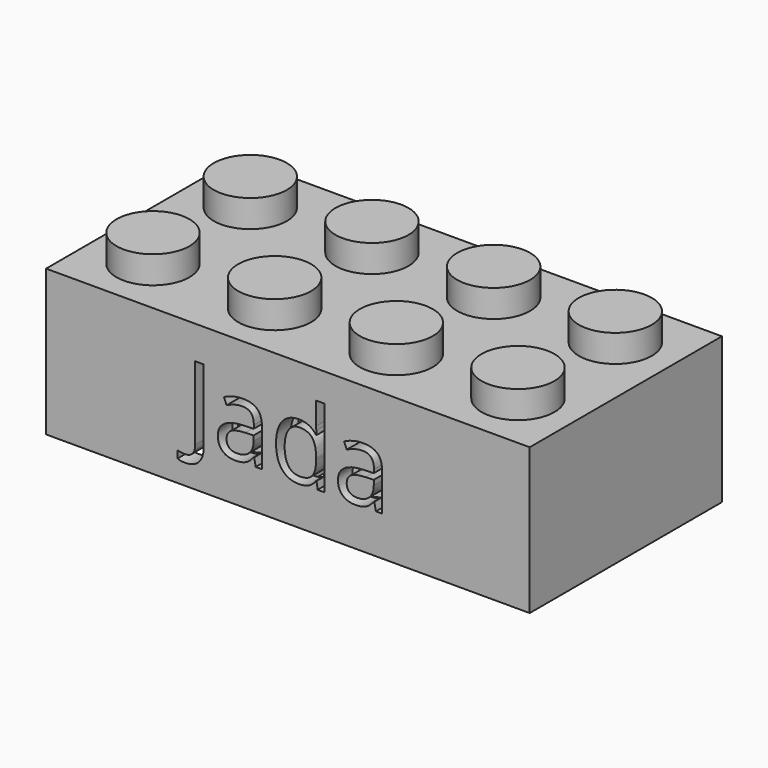
from build123d import *

# Parameters (mm, degrees)
F0_W          = 31.8
F0_H          = 15.8
F1_DEPTH      = 9.6
F2_W          = 29.4
F2_H          = 13.4
F3_DEPTH      = 8.4
F4_R          = 2.4
F5_DEPTH      = 1.8
F6_R          = 1.3
F7_DEPTH      = 1.2
F8_R          = 3.255
F8_R_2        = 2.4
F9_DEPTH      = 8.4
F10_W         = 0.6
F10_H         = 0.3
F11_DEPTH     = 8.4
F12_W         = 0.3
F12_H         = 0.6
F13_DEPTH     = 8.4
F14_W         = 0.6
F14_H         = 4
F15_DEPTH     = 6.4
F16_W         = 0.6
F16_H         = 4
F17_DEPTH     = 6.4
F18_TEXT_SIZE = 6.759243681
F19_DEPTH     = 1.2


# Not quite as in the source:
# - Text() gives the source's letters only with a copy of the font that has no kerning and outlines rounded to 1/6400 em; it was checked with that copy


with BuildPart() as f1:
    # F0 (on Top) → F1 (new body)
    with BuildSketch(Plane.XY):
        Rectangle(F0_W, F0_H)
    extrude(amount=F1_DEPTH)

    # F2 (on face) → F3 (cut)
    with BuildSketch(Plane(origin=(0, 0, 0), x_dir=(1, 0, 0), z_dir=(0, 0, -1))):
        Rectangle(F2_W, F2_H)
    extrude(amount=-F3_DEPTH, mode=Mode.SUBTRACT)

    # F4 (on face) → F5 (join)
    with BuildSketch(Plane.XY.offset(9.6)):
        with Locations((-11.95, 3.95)):
            Circle(F4_R)
        with Locations((-11.95, -4.05)):
            Circle(F4_R)
        with Locations((-3.95, 3.95)):
            Circle(F4_R)
        with Locations((-3.95, -4.05)):
            Circle(F4_R)
        with Locations((4.05, 3.95)):
            Circle(F4_R)
        with Locations((4.05, -4.05)):
            Circle(F4_R)
        with Locations((12.05, 3.95)):
            Circle(F4_R)
        with Locations((12.05, -4.05)):
            Circle(F4_R)
    extrude(amount=F5_DEPTH)

    # F6 (on face) → F7 (cut)
    with BuildSketch(Plane(origin=(0, 0, 8.4), x_dir=(1, 0, 0), z_dir=(0, 0, -1))):
        with Locations((-11.95, 3.95)):
            Circle(F6_R)
        with Locations((-11.95, -4.05)):
            Circle(F6_R)
        with Locations((-3.95, 3.95)):
            Circle(F6_R)
        with Locations((-3.95, -4.05)):
            Circle(F6_R)
        with Locations((4.05, 3.95)):
            Circle(F6_R)
        with Locations((4.05, -4.05)):
            Circle(F6_R)
        with Locations((12.05, 3.95)):
            Circle(F6_R)
        with Locations((12.05, -4.05)):
            Circle(F6_R)
    extrude(amount=-F7_DEPTH, mode=Mode.SUBTRACT)

    # F8 (on face) → F9 (join, through all)
    with BuildSketch(Plane(origin=(0, 0, 8.4), x_dir=(1, 0, 0), z_dir=(0, 0, -1))):
        with Locations((-7.95, -0.05)):
            Circle(F8_R)
        with Locations((-7.95, -0.05)):
            Circle(F8_R_2, mode=Mode.SUBTRACT)
        with Locations((0.05, -0.05)):
            Circle(F8_R)
        with Locations((0.05, -0.05)):
            Circle(F8_R_2, mode=Mode.SUBTRACT)
        with Locations((8.05, -0.05)):
            Circle(F8_R)
        with Locations((8.05, -0.05)):
            Circle(F8_R_2, mode=Mode.SUBTRACT)
    extrude(amount=F9_DEPTH)

    # F10 (on face) → F11 (join, through all)
    with BuildSketch(Plane(origin=(0, 0, 0), x_dir=(1, 0, 0), z_dir=(0, 0, -1))):
        with Locations((-11.95, 6.55)):
            Rectangle(F10_W, F10_H)
        with Locations((-11.95, -6.55)):
            Rectangle(F10_W, F10_H)
        with Locations((-3.95, 6.55)):
            Rectangle(F10_W, F10_H)
        with Locations((-3.95, -6.55)):
            Rectangle(F10_W, F10_H)
        with Locations((4.05, 6.55)):
            Rectangle(F10_W, F10_H)
        with Locations((4.05, -6.55)):
            Rectangle(F10_W, F10_H)
        with Locations((12.05, 6.55)):
            Rectangle(F10_W, F10_H)
        with Locations((12.05, -6.55)):
            Rectangle(F10_W, F10_H)
    extrude(amount=-F11_DEPTH)

    # F12 (on face) → F13 (join, through all)
    with BuildSketch(Plane(origin=(0, 0, 0), x_dir=(1, 0, 0), z_dir=(0, 0, -1))):
        with Locations((-14.55, 3.95)):
            Rectangle(F12_W, F12_H)
        with Locations((-14.55, -4.05)):
            Rectangle(F12_W, F12_H)
        with Locations((14.55, 3.95)):
            Rectangle(F12_W, F12_H)
        with Locations((14.55, -4.05)):
            Rectangle(F12_W, F12_H)
    extrude(amount=-F13_DEPTH)

    # F14 (on face) → F15 (join)
    with BuildSketch(Plane(origin=(0, 0, 8.4), x_dir=(1, 0, 0), z_dir=(0, 0, -1))):
        with Locations((0.05, 4.956481047)):
            Rectangle(F14_W, F14_H)
    extrude(amount=F15_DEPTH)

    # F16 (on face) → F17 (join)
    with BuildSketch(Plane(origin=(0, 0, 8.4), x_dir=(1, 0, 0), z_dir=(0, 0, -1))):
        with Locations((0.05, -5.093377782)):
            Rectangle(F16_W, F16_H)
    extrude(amount=F17_DEPTH)

    # F18 (on face) → F19 (cut)
    with BuildSketch(Plane.XZ.offset(7.9)):
        with Locations((-6.722807133, 2.6020971127)):
            Text('Jada', F18_TEXT_SIZE, font='Open Sans', text_align=(TextAlign.LEFT, TextAlign.BOTTOM))
    extrude(amount=-F19_DEPTH, mode=Mode.SUBTRACT)


solid = f1.part
